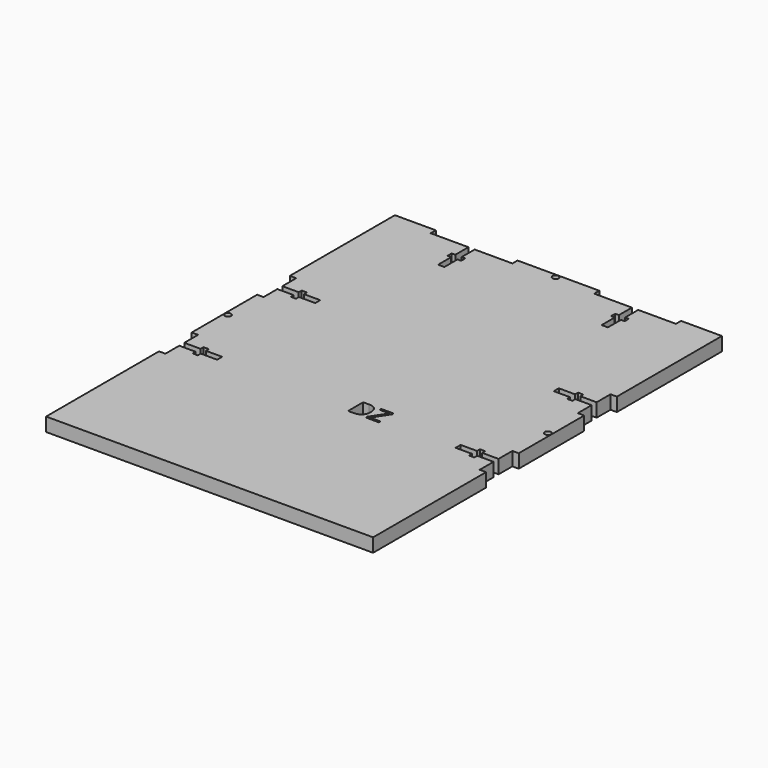
from build123d import *

# Parameters (mm, degrees)
F0_R     = 1.4605
F1_DEPTH = 6.35


# Not quite as in the source:
# - a feature names something its author has since deleted; it is built from what else it names


with BuildPart() as f1:
    # F0 (on Top) → F1 (new body)
    with BuildSketch(Plane.XY):
        Polygon((-57.1500000004, 101.5999999999), (-76.2, 101.5999999999), (-76.2, 40.4022223395), (-73.2282, 40.4022223395), (-73.2282, 32.3377223395), (-65.6082, 32.3377223395), (-65.6082, 34.0522223395), (-63.1952, 34.0522223395), (-63.1952, 32.3377223395), (-55.5752, 32.3377223395), (-55.5752, 30.8772223395), (-55.5752, 29.4167223395), (-63.1952, 29.4167223395), (-63.1952, 27.7022223395), (-65.6082, 27.7022223395), (-65.6082, 29.4167223395), (-73.2282, 29.4167223395), (-73.2282, 21.3522223395), (-76.2, 21.3522223395), (-76.2, -16.7477776605), (-73.2282, -16.7477776605), (-73.2282, -24.8122776605), (-65.6082, -24.8122776605), (-65.6082, -23.0977776605), (-63.1952, -23.0977776605), (-63.1952, -24.8122776605), (-55.5752, -24.8122776605), (-55.5752, -26.2727776605), (-55.5752, -27.7332776605), (-63.1952, -27.7332776605), (-63.1952, -29.4477776605), (-65.6082, -29.4477776605), (-65.6082, -27.7332776605), (-73.2282, -27.7332776605), (-73.2282, -35.7977776604), (-76.2, -35.7977776604), (-76.2, -101.5999999999), (76.2, -101.5999999999), (76.2, -35.7977776604), (73.2282, -35.7977776604), (73.2282, -27.7332776605), (65.6082, -27.7332776605), (65.6082, -29.4477776605), (63.1952, -29.4477776605), (63.1952, -27.7332776605), (55.5752, -27.7332776605), (55.5752, -26.2727776605), (55.5752, -24.8122776605), (63.1952, -24.8122776605), (63.1952, -23.0977776605), (65.6082, -23.0977776605), (65.6082, -24.8122776605), (73.2282, -24.8122776605), (73.2282, -16.7477776605), (76.2, -16.7477776605), (76.2, 21.3522223395), (73.2282, 21.3522223395), (73.2282, 29.4167223395), (65.6082, 29.4167223395), (65.6082, 27.7022223395), (63.1952, 27.7022223395), (63.1952, 29.4167223395), (55.5752, 29.4167223395), (55.5752, 30.8772223395), (55.5752, 32.3377223395), (63.1952, 32.3377223395), (63.1952, 34.0522223395), (65.6082, 34.0522223395), (65.6082, 32.3377223395), (73.2282, 32.3377223395), (73.2282, 40.4022223395), (76.2, 40.4022223395), (76.2, 101.5999999999), (57.1499999998, 101.5999999999), (57.1499999998, 98.6281999999), (39.5605000002, 98.6281999999), (39.5605000002, 91.0081999999), (41.2750000002, 91.0081999999), (41.2750000002, 88.5951999999), (39.5605000002, 88.5951999999), (39.5605000002, 80.9751999999), (38.1000000002, 80.9751999999), (36.6395000002, 80.9751999999), (36.6395000002, 88.5951999999), (34.9250000002, 88.5951999999), (34.9250000002, 91.0081999999), (36.6395000002, 91.0081999999), (36.6395000002, 98.6281999999), (19.05, 98.6281999999), (19.05, 101.5999999999), (-19.05, 101.5999999999), (-19.05, 98.6281999999), (-21.3974503974, 98.6281999999), (-36.6395000002, 98.6281999999), (-36.6395000002, 91.0081999999), (-34.9250000002, 91.0081999999), (-34.9250000002, 88.5951999999), (-36.6395000002, 88.5951999999), (-36.6395000002, 80.9751999999), (-38.1000000002, 80.9751999999), (-39.5605000002, 80.9751999999), (-39.5605000002, 88.5951999999), (-41.2750000002, 88.5951999999), (-41.2750000002, 91.0081999999), (-39.5605000002, 91.0081999999), (-39.5605000002, 98.6281999999), (-57.1500000004, 98.6281999999), align=None)
        with BuildLine():
            add(Edge.make_bspline(
                [(12.7658935974, -21.8633876268), (13.9035680881, -23.0010621174), (13.9035680881, -25.0432889762)],
                knots=[0, 0, 0, 1, 1, 1], degree=2))
            add(Edge.make_bspline(
                [(13.9035680881, -25.0432889762), (13.9035680881, -27.2223065019), (12.7206178133, -28.3753940255)],
                knots=[0, 0, 0, 1, 1, 1], degree=2))
            add(Edge.make_bspline(
                [(12.7206178133, -28.3753940255), (11.5376675385, -29.5284815491), (9.3162641723, -29.5284815491)],
                knots=[0, 0, 0, 1, 1, 1], degree=2))
            Line((9.3162641723, -29.5284815491), (6.8771517165, -29.5284815491))
            Line((6.8771517165, -29.5284815491), (6.8771517165, -20.7257131361))
            Line((6.8771517165, -20.7257131361), (9.5744324733, -20.7257131361))
            add(Edge.make_bspline(
                [(9.5744324733, -20.7257131361), (11.6282191068, -20.7257131361), (12.7658935974, -21.8633876268)],
                knots=[0, 0, 0, 1, 1, 1], degree=2))
        make_face(mode=Mode.SUBTRACT)
        Polygon((21.2016391646, -28.6017729462), (21.2016391646, -29.5284815491), (15.1500971236, -29.5284815491), (15.1500971236, -28.7270038385), (19.8221727203, -21.6466418517), (15.294594307, -21.6466418517), (15.294594307, -20.7257131361), (21.0687017558, -20.7257131361), (21.0687017558, -21.5271908467), (16.3966261591, -28.6017729462), align=None, mode=Mode.SUBTRACT)
        with Locations((-74.5805352926, 2.3022223395)):
            Circle(F0_R, mode=Mode.SUBTRACT)
        with Locations((74.5805352926, 2.3022223395)):
            Circle(F0_R, mode=Mode.SUBTRACT)
        with Locations((0, 100.0089123845)):
            Circle(F0_R, mode=Mode.SUBTRACT)
    extrude(amount=F1_DEPTH)


solid = f1.part
